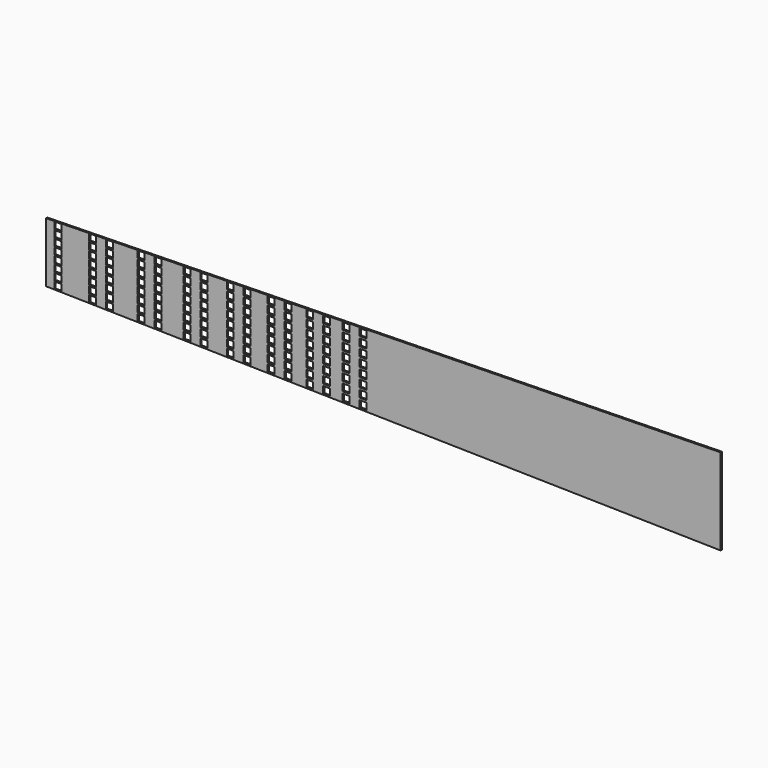
from build123d import *

# Parameters (mm, degrees)
F0_W     = 6.5
F0_H     = 6.5
F1_DEPTH = 1.524
F3_R     = 1.1303
F4_DEPTH = 1001


# Not quite as in the source:
# - an extrude ends at something that could not be found from the text; its depth is read off the source's solid


with BuildPart() as f1:
    # F0 (on Front) → F1 (new body)
    with BuildSketch(Plane.XZ):
        Polygon((0, 56.388), (0, 0), (304.8, -5.97408), (304.8, 62.36208), align=None)
        with Locations((43.7079136, 2.7746592818)):
            Rectangle(F0_W, F0_H, mode=Mode.SUBTRACT)
        with Locations((59.5829136, 2.5024030318)):
            Rectangle(F0_W, F0_H, mode=Mode.SUBTRACT)
        with Locations((11.1125, 3.333670625)):
            Rectangle(F0_W, F0_H, mode=Mode.SUBTRACT)
        with Locations((89.4571236, 1.9900603303)):
            Rectangle(F0_W, F0_H, mode=Mode.SUBTRACT)
        with Locations((105.3321236, 1.7178040803)):
            Rectangle(F0_W, F0_H, mode=Mode.SUBTRACT)
        with Locations((132.6397144, 1.249478898)):
            Rectangle(F0_W, F0_H, mode=Mode.SUBTRACT)
        with Locations((148.5147144, 0.977222648)):
            Rectangle(F0_W, F0_H, mode=Mode.SUBTRACT)
        with Locations((173.3904076, 0.5506045097)):
            Rectangle(F0_W, F0_H, mode=Mode.SUBTRACT)
        with Locations((189.2654076, 0.2783482597)):
            Rectangle(F0_W, F0_H, mode=Mode.SUBTRACT)
        with Locations((211.8689692, -0.1093028218)):
            Rectangle(F0_W, F0_H, mode=Mode.SUBTRACT)
        with Locations((227.7439692, -0.3815590718)):
            Rectangle(F0_W, F0_H, mode=Mode.SUBTRACT)
        with Locations((227.7439692, 7.7896209282)):
            Rectangle(F0_W, F0_H, mode=Mode.SUBTRACT)
        with Locations((248.1798948, -0.7320351958)):
            Rectangle(F0_W, F0_H, mode=Mode.SUBTRACT)
        with Locations((264.0548948, -1.0042914458)):
            Rectangle(F0_W, F0_H, mode=Mode.SUBTRACT)
        with Locations((282.453588, -1.3198290342)):
            Rectangle(F0_W, F0_H, mode=Mode.SUBTRACT)
        with Locations((298.328588, -1.5920852842)):
            Rectangle(F0_W, F0_H, mode=Mode.SUBTRACT)
        with Locations((248.1798948, 7.5559848042)):
            Rectangle(F0_W, F0_H, mode=Mode.SUBTRACT)
        with Locations((264.0548948, 7.3446885542)):
            Rectangle(F0_W, F0_H, mode=Mode.SUBTRACT)
        with Locations((282.453588, 7.1358309658)):
            Rectangle(F0_W, F0_H, mode=Mode.SUBTRACT)
        with Locations((298.328588, 6.9270747158)):
            Rectangle(F0_W, F0_H, mode=Mode.SUBTRACT)
        with Locations((11.1125, 10.430670625)):
            Rectangle(F0_W, F0_H, mode=Mode.SUBTRACT)
        with Locations((43.7079136, 10.0619192818)):
            Rectangle(F0_W, F0_H, mode=Mode.SUBTRACT)
        with Locations((59.5829136, 9.8506230318)):
            Rectangle(F0_W, F0_H, mode=Mode.SUBTRACT)
        with Locations((11.1125, 17.527670625)):
            Rectangle(F0_W, F0_H, mode=Mode.SUBTRACT)
        with Locations((43.7079136, 17.3491792818)):
            Rectangle(F0_W, F0_H, mode=Mode.SUBTRACT)
        with Locations((59.5829136, 17.1988430318)):
            Rectangle(F0_W, F0_H, mode=Mode.SUBTRACT)
        with Locations((89.4571236, 9.5008403303)):
            Rectangle(F0_W, F0_H, mode=Mode.SUBTRACT)
        with Locations((105.3321236, 9.2895440803)):
            Rectangle(F0_W, F0_H, mode=Mode.SUBTRACT)
        with Locations((132.6397144, 8.971078898)):
            Rectangle(F0_W, F0_H, mode=Mode.SUBTRACT)
        with Locations((148.5147144, 8.762322648)):
            Rectangle(F0_W, F0_H, mode=Mode.SUBTRACT)
        with Locations((89.4571236, 17.0116203303)):
            Rectangle(F0_W, F0_H, mode=Mode.SUBTRACT)
        with Locations((105.3321236, 16.8612840803)):
            Rectangle(F0_W, F0_H, mode=Mode.SUBTRACT)
        with Locations((132.6397144, 16.692678898)):
            Rectangle(F0_W, F0_H, mode=Mode.SUBTRACT)
        with Locations((148.5147144, 16.547422648)):
            Rectangle(F0_W, F0_H, mode=Mode.SUBTRACT)
        with Locations((11.1125, 24.624670625)):
            Rectangle(F0_W, F0_H, mode=Mode.SUBTRACT)
        with Locations((43.7079136, 24.6364392818)):
            Rectangle(F0_W, F0_H, mode=Mode.SUBTRACT)
        with Locations((59.5829136, 24.5470630318)):
            Rectangle(F0_W, F0_H, mode=Mode.SUBTRACT)
        with Locations((89.4571236, 24.5224003303)):
            Rectangle(F0_W, F0_H, mode=Mode.SUBTRACT)
        with Locations((105.3321236, 24.4330240803)):
            Rectangle(F0_W, F0_H, mode=Mode.SUBTRACT)
        with Locations((132.6397144, 24.414278898)):
            Rectangle(F0_W, F0_H, mode=Mode.SUBTRACT)
        with Locations((148.5147144, 24.332522648)):
            Rectangle(F0_W, F0_H, mode=Mode.SUBTRACT)
        with Locations((173.3904076, 8.4728645097)):
            Rectangle(F0_W, F0_H, mode=Mode.SUBTRACT)
        with Locations((189.2654076, 8.2615682597)):
            Rectangle(F0_W, F0_H, mode=Mode.SUBTRACT)
        with Locations((211.8689692, 8.0009171782)):
            Rectangle(F0_W, F0_H, mode=Mode.SUBTRACT)
        with Locations((173.3904076, 16.3951245097)):
            Rectangle(F0_W, F0_H, mode=Mode.SUBTRACT)
        with Locations((189.2654076, 16.2447882597)):
            Rectangle(F0_W, F0_H, mode=Mode.SUBTRACT)
        with Locations((211.8689692, 16.1111371782)):
            Rectangle(F0_W, F0_H, mode=Mode.SUBTRACT)
        with Locations((227.7439692, 15.9608009282)):
            Rectangle(F0_W, F0_H, mode=Mode.SUBTRACT)
        with Locations((248.1798948, 15.8440048042)):
            Rectangle(F0_W, F0_H, mode=Mode.SUBTRACT)
        with Locations((264.0548948, 15.6936685542)):
            Rectangle(F0_W, F0_H, mode=Mode.SUBTRACT)
        with Locations((298.328588, 15.4462347158)):
            Rectangle(F0_W, F0_H, mode=Mode.SUBTRACT)
        with Locations((282.453588, 15.5914909658)):
            Rectangle(F0_W, F0_H, mode=Mode.SUBTRACT)
        with Locations((173.3904076, 24.3173845097)):
            Rectangle(F0_W, F0_H, mode=Mode.SUBTRACT)
        with Locations((189.2654076, 24.2280082597)):
            Rectangle(F0_W, F0_H, mode=Mode.SUBTRACT)
        with Locations((211.8689692, 24.2213571782)):
            Rectangle(F0_W, F0_H, mode=Mode.SUBTRACT)
        with Locations((227.7439692, 24.1319809282)):
            Rectangle(F0_W, F0_H, mode=Mode.SUBTRACT)
        with Locations((248.1798948, 24.1320248042)):
            Rectangle(F0_W, F0_H, mode=Mode.SUBTRACT)
        with Locations((264.0548948, 24.0426485542)):
            Rectangle(F0_W, F0_H, mode=Mode.SUBTRACT)
        with Locations((282.453588, 24.0471509658)):
            Rectangle(F0_W, F0_H, mode=Mode.SUBTRACT)
        with Locations((298.328588, 23.9653947158)):
            Rectangle(F0_W, F0_H, mode=Mode.SUBTRACT)
        with Locations((11.1125, 31.721670625)):
            Rectangle(F0_W, F0_H, mode=Mode.SUBTRACT)
        with Locations((43.7079136, 31.9236992818)):
            Rectangle(F0_W, F0_H, mode=Mode.SUBTRACT)
        with Locations((59.5829136, 31.8952830318)):
            Rectangle(F0_W, F0_H, mode=Mode.SUBTRACT)
        with Locations((89.4571236, 32.0331803303)):
            Rectangle(F0_W, F0_H, mode=Mode.SUBTRACT)
        with Locations((105.3321236, 32.0047640803)):
            Rectangle(F0_W, F0_H, mode=Mode.SUBTRACT)
        with Locations((132.6397144, 32.135878898)):
            Rectangle(F0_W, F0_H, mode=Mode.SUBTRACT)
        with Locations((148.5147144, 32.117622648)):
            Rectangle(F0_W, F0_H, mode=Mode.SUBTRACT)
        with Locations((11.1125, 38.818670625)):
            Rectangle(F0_W, F0_H, mode=Mode.SUBTRACT)
        with Locations((43.7079136, 39.2109592818)):
            Rectangle(F0_W, F0_H, mode=Mode.SUBTRACT)
        with Locations((59.5829136, 39.2435030318)):
            Rectangle(F0_W, F0_H, mode=Mode.SUBTRACT)
        with Locations((11.1125, 45.915670625)):
            Rectangle(F0_W, F0_H, mode=Mode.SUBTRACT)
        with Locations((43.7079136, 46.4982192818)):
            Rectangle(F0_W, F0_H, mode=Mode.SUBTRACT)
        with Locations((59.5829136, 46.5917230318)):
            Rectangle(F0_W, F0_H, mode=Mode.SUBTRACT)
        with Locations((89.4571236, 39.5439603303)):
            Rectangle(F0_W, F0_H, mode=Mode.SUBTRACT)
        with Locations((105.3321236, 39.5765040803)):
            Rectangle(F0_W, F0_H, mode=Mode.SUBTRACT)
        with Locations((132.6397144, 39.857478898)):
            Rectangle(F0_W, F0_H, mode=Mode.SUBTRACT)
        with Locations((148.5147144, 39.902722648)):
            Rectangle(F0_W, F0_H, mode=Mode.SUBTRACT)
        with Locations((89.4571236, 47.0547403303)):
            Rectangle(F0_W, F0_H, mode=Mode.SUBTRACT)
        with Locations((105.3321236, 47.1482440803)):
            Rectangle(F0_W, F0_H, mode=Mode.SUBTRACT)
        with Locations((132.6397144, 47.579078898)):
            Rectangle(F0_W, F0_H, mode=Mode.SUBTRACT)
        with Locations((148.5147144, 47.687822648)):
            Rectangle(F0_W, F0_H, mode=Mode.SUBTRACT)
        with Locations((173.3904076, 32.2396445097)):
            Rectangle(F0_W, F0_H, mode=Mode.SUBTRACT)
        with Locations((189.2654076, 32.2112282597)):
            Rectangle(F0_W, F0_H, mode=Mode.SUBTRACT)
        with Locations((211.8689692, 32.3315771782)):
            Rectangle(F0_W, F0_H, mode=Mode.SUBTRACT)
        with Locations((227.7439692, 32.3031609282)):
            Rectangle(F0_W, F0_H, mode=Mode.SUBTRACT)
        with Locations((248.1798948, 32.4200448042)):
            Rectangle(F0_W, F0_H, mode=Mode.SUBTRACT)
        with Locations((264.0548948, 32.3916285542)):
            Rectangle(F0_W, F0_H, mode=Mode.SUBTRACT)
        with Locations((282.453588, 32.5028109658)):
            Rectangle(F0_W, F0_H, mode=Mode.SUBTRACT)
        with Locations((298.328588, 32.4845547158)):
            Rectangle(F0_W, F0_H, mode=Mode.SUBTRACT)
        with Locations((173.3904076, 40.1619045097)):
            Rectangle(F0_W, F0_H, mode=Mode.SUBTRACT)
        with Locations((189.2654076, 40.1944482597)):
            Rectangle(F0_W, F0_H, mode=Mode.SUBTRACT)
        with Locations((211.8689692, 40.4417971782)):
            Rectangle(F0_W, F0_H, mode=Mode.SUBTRACT)
        with Locations((227.7439692, 40.4743409282)):
            Rectangle(F0_W, F0_H, mode=Mode.SUBTRACT)
        with Locations((173.3904076, 48.0841645097)):
            Rectangle(F0_W, F0_H, mode=Mode.SUBTRACT)
        with Locations((189.2654076, 48.1776682597)):
            Rectangle(F0_W, F0_H, mode=Mode.SUBTRACT)
        with Locations((248.1798948, 40.7080648042)):
            Rectangle(F0_W, F0_H, mode=Mode.SUBTRACT)
        with Locations((264.0548948, 40.7406085542)):
            Rectangle(F0_W, F0_H, mode=Mode.SUBTRACT)
        with Locations((282.453588, 40.9584709658)):
            Rectangle(F0_W, F0_H, mode=Mode.SUBTRACT)
        with Locations((298.328588, 41.0037147158)):
            Rectangle(F0_W, F0_H, mode=Mode.SUBTRACT)
        with Locations((11.1125, 53.012670625)):
            Rectangle(F0_W, F0_H, mode=Mode.SUBTRACT)
        with Locations((43.7079136, 53.7854792818)):
            Rectangle(F0_W, F0_H, mode=Mode.SUBTRACT)
        with Locations((59.5829136, 53.9399430318)):
            Rectangle(F0_W, F0_H, mode=Mode.SUBTRACT)
        with Locations((89.4571236, 54.5655203303)):
            Rectangle(F0_W, F0_H, mode=Mode.SUBTRACT)
        with Locations((105.3321236, 54.7199840803)):
            Rectangle(F0_W, F0_H, mode=Mode.SUBTRACT)
        with Locations((132.6397144, 55.300678898)):
            Rectangle(F0_W, F0_H, mode=Mode.SUBTRACT)
        with Locations((148.5147144, 55.472922648)):
            Rectangle(F0_W, F0_H, mode=Mode.SUBTRACT)
        with Locations((211.8689692, 48.5520171782)):
            Rectangle(F0_W, F0_H, mode=Mode.SUBTRACT)
        with Locations((227.7439692, 48.6455209282)):
            Rectangle(F0_W, F0_H, mode=Mode.SUBTRACT)
        with Locations((173.3904076, 56.0064245097)):
            Rectangle(F0_W, F0_H, mode=Mode.SUBTRACT)
        with Locations((189.2654076, 56.1608882597)):
            Rectangle(F0_W, F0_H, mode=Mode.SUBTRACT)
        with Locations((211.8689692, 56.6622371782)):
            Rectangle(F0_W, F0_H, mode=Mode.SUBTRACT)
        with Locations((227.7439692, 56.8167009282)):
            Rectangle(F0_W, F0_H, mode=Mode.SUBTRACT)
        with Locations((248.1798948, 48.9960848042)):
            Rectangle(F0_W, F0_H, mode=Mode.SUBTRACT)
        with Locations((264.0548948, 49.0895885542)):
            Rectangle(F0_W, F0_H, mode=Mode.SUBTRACT)
        with Locations((282.453588, 49.4141309658)):
            Rectangle(F0_W, F0_H, mode=Mode.SUBTRACT)
        with Locations((298.328588, 49.5228747158)):
            Rectangle(F0_W, F0_H, mode=Mode.SUBTRACT)
        with Locations((248.1798948, 57.2841048042)):
            Rectangle(F0_W, F0_H, mode=Mode.SUBTRACT)
        with Locations((264.0548948, 57.4385685542)):
            Rectangle(F0_W, F0_H, mode=Mode.SUBTRACT)
        with Locations((282.453588, 57.8697909658)):
            Rectangle(F0_W, F0_H, mode=Mode.SUBTRACT)
        with Locations((298.328588, 58.0420347158)):
            Rectangle(F0_W, F0_H, mode=Mode.SUBTRACT)
        Polygon((304.8, 62.36208), (304.8, -5.97408), (635, -12.446), (635, 68.834), align=None)
    extrude(amount=F1_DEPTH)

    # F3 (on face) → F4 (cut, through all)
    with BuildSketch(Plane.XZ.offset(1.524)):
        with Locations((97.3946236, 8.0847413075)):
            Circle(F3_R)
        with Locations((3.175, 8.1216754)):
            Circle(F3_R)
        with Locations((181.3279076, 8.0518394602)):
            Circle(F3_R)
        with Locations((290.391088, 8.0090866935)):
            Circle(F3_R)
        with Locations((409.2984448, 7.9624750096)):
            Circle(F3_R)
        with Locations((524.05534, 7.9174903067)):
            Circle(F3_R)
        with Locations((624.435886, 7.8781411327)):
            Circle(F3_R)
        with Locations((97.3946236, 48.3032586925)):
            Circle(F3_R)
        with Locations((3.175, 48.2663246)):
            Circle(F3_R)
        with Locations((181.3279076, 48.3361605398)):
            Circle(F3_R)
        with Locations((290.391088, 48.3789133065)):
            Circle(F3_R)
        with Locations((409.2984448, 48.4255249904)):
            Circle(F3_R)
        with Locations((524.05534, 48.4705096933)):
            Circle(F3_R)
        with Locations((624.435886, 48.5098588673)):
            Circle(F3_R)
    extrude(amount=F4_DEPTH, mode=Mode.SUBTRACT)


solid = f1.part
